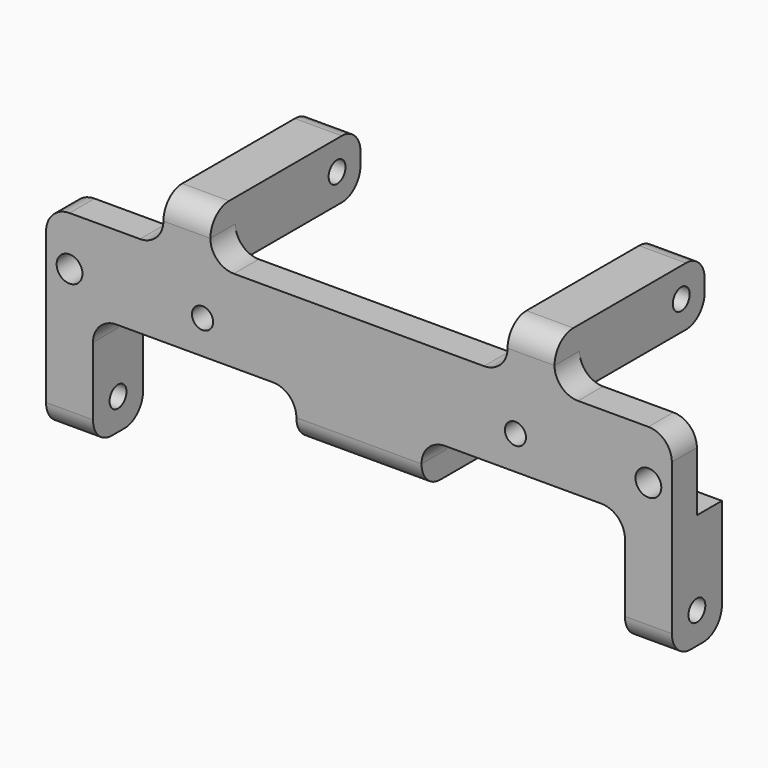
from build123d import *

# Parameters (mm, degrees)
F0_R      = 1.65
F1_DEPTH  = 4
F2_W      = 6
F2_H      = 14.7
F2_W_2    = 16
F2_H_2    = 6
F3_DEPTH  = 4
F4_W      = 6
F4_H      = 6
F5_DEPTH  = 20
F6_DEPTH  = 1.5
F7_DEPTH  = 11
F8_R      = 1.65
F9_DEPTH  = 14.701
F10_R     = 1.35
F11_DEPTH = 80.001
F12_R     = 1.35
F13_DEPTH = 65.001
F14_R     = 2.99999
F15_R     = 1.35
F16_DEPTH = 24.001


# Not quite as in the source:
# - a fillet or chamfer is up to 0.001 mm smaller than in the source, because OpenCascade refuses the exact size


with BuildPart() as f1:
    # F0 (on Front) → F1 (new body)
    with BuildSketch(Plane.XZ):
        Polygon((-25, 6.3), (-40, 6.3), (-40, -4.3), (-40, -19), (-34, -19), (-34, -4.3), (-8, -4.3), (-8, -10.3), (8, -10.3), (8, -4.3), (34, -4.3), (34, -19), (40, -19), (40, -4.3), (40, 6.3), (25, 6.3), (25, 12.3), (19, 12.3), (19, 6.3), (-19, 6.3), (-19, 12.3), (-25, 12.3), align=None)
        with Locations((-37, 0)):
            Circle(F0_R, mode=Mode.SUBTRACT)
        with Locations((37, 0)):
            Circle(F0_R, mode=Mode.SUBTRACT)
    extrude(amount=F1_DEPTH)

    # F2 (on face) → F3 (join)
    with BuildSketch(Plane(origin=(0, 0, 0), x_dir=(-1, 0, 0), z_dir=(0, 1, 0))):
        with Locations((37, -11.65)):
            Rectangle(F2_W, F2_H)
        with Locations((0, -7.3)):
            Rectangle(F2_W_2, F2_H_2)
        with Locations((-37, -11.65)):
            Rectangle(F2_W, F2_H)
    extrude(amount=F3_DEPTH)

    # F4 (on face) → F5 (join)
    with BuildSketch(Plane(origin=(0, 0, 0), x_dir=(-1, 0, 0), z_dir=(0, 1, 0))):
        with Locations((-22, 9.3)):
            Rectangle(F4_W, F4_H)
        with Locations((22, 9.3)):
            Rectangle(F4_W, F4_H)
    extrude(amount=F5_DEPTH)

    # F6 (add): faces of the model
    f6_faces = [f1.faces().sort_by_distance(p)[0] for p in [
        (22, 10, 6.3),
        (-22, 10, 6.3),
    ]]
    extrude(f6_faces, amount=F6_DEPTH)

    # F7 (add): a face of the model
    f7_faces = [f1.faces().sort_by_distance(p)[0] for p in [
        (0, 4, -7.3),
    ]]
    extrude(f7_faces, amount=F7_DEPTH)

    # F8 (on face) → F9 (cut, through all)
    with BuildSketch(Plane.XY.offset(-4.3)):
        with Locations((5, 12)):
            Circle(F8_R)
        with Locations((-5, 12)):
            Circle(F8_R)
    extrude(amount=-F9_DEPTH, mode=Mode.SUBTRACT)

    # F10 (on face) → F11 (cut, through all)
    with BuildSketch(Plane.YZ.offset(40)):
        with Locations((0, -15)):
            Circle(F10_R)
    extrude(amount=-F11_DEPTH, mode=Mode.SUBTRACT)

    # F12 (on face) → F13 (cut, through all)
    with BuildSketch(Plane(origin=(-25, 0, 0), x_dir=(0, -1, 0), z_dir=(-1, 0, 0))):
        with Locations((-16.25, 8.55)):
            Circle(F12_R)
    extrude(amount=-F13_DEPTH, mode=Mode.SUBTRACT)

    # F14 (radius 3 in the source; OpenCascade refuses exactly that, so slightly less here)
    f14_edges = [f1.edges().sort_by_distance(p)[0] for p in [
        (-37, -4, -19),
        (37, -4, -19),
        (37, 4, -19),
        (-37, 4, -19),
        (8, 15, -7.3),
        (-8, 15, -7.3),
        (-22, 20, 12.3),
        (22, 20, 12.3),
        (-22, 20, 4.8),
        (22, 20, 4.8),
        (-22, -4, 12.3),
        (22, -4, 12.3),
        (-34, -2, -4.3),
        (34, -2, -4.3),
        (-8, -2, -4.3),
        (8, -2, -4.3),
        (-25, -2, 6.3),
        (19, -2, 6.3),
        (-19, -2, 6.3),
        (25, -2, 6.3),
        (-40, -2, 6.3),
        (40, -2, 6.3),
        (0, -4, -10.3),
    ]]
    fillet(f14_edges, radius=F14_R)

    # F15 (on face) → F16 (cut, through all)
    with BuildSketch(Plane.XZ.offset(4)):
        with Locations((-20, 0)):
            Circle(F15_R)
        with Locations((20, 0)):
            Circle(F15_R)
    extrude(amount=-F16_DEPTH, mode=Mode.SUBTRACT)


solid = f1.part
